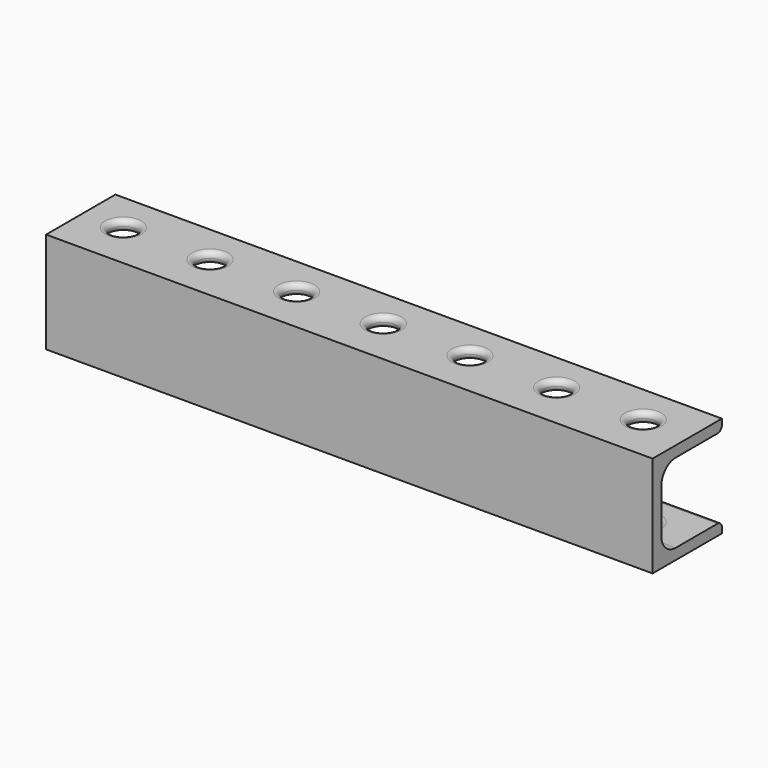
from build123d import *

# Parameters (mm, degrees)
F1_DEPTH = 168
F2_R     = 3.5
F3_DEPTH = 33
F4_R     = 5
F5_R     = 1.5
F6_R     = 1.49999
F7_R     = 1.49999
F8_R     = 1.49999


# Not quite as in the source:
# - a fillet or chamfer is up to 0.001 mm smaller than in the source, because OpenCascade refuses the exact size


with BuildPart() as f1:
    # F0 (on Right) → F1 (new body)
    with BuildSketch(Plane.YZ):
        Polygon((24, 27.9123237882), (0, 27.9123237882), (0, 0), (0, -0.0876762118), (24, -0.0876762118), (24, 2.9123237882), (3, 2.9123237882), (3, 24.9123237882), (24, 24.9123237882), align=None)
    extrude(amount=F1_DEPTH)

    # F2 (on face) → F3 (cut)
    with BuildSketch(Plane.XY.offset(27.9123237882)):
        with Locations((11, 13)):
            Circle(F2_R)
        with Locations((35, 13)):
            Circle(F2_R)
        with Locations((59, 13)):
            Circle(F2_R)
        with Locations((83, 13)):
            Circle(F2_R)
        with Locations((107, 13)):
            Circle(F2_R)
        with Locations((131, 13)):
            Circle(F2_R)
        with Locations((155, 13)):
            Circle(F2_R)
    extrude(amount=-F3_DEPTH, mode=Mode.SUBTRACT)

    # F4
    f4_edges = [f1.edges().sort_by_distance(p)[0] for p in [
        (84, 3, 24.912324),
        (84, 3, 2.912324),
    ]]
    fillet(f4_edges, radius=F4_R)

    # F5
    f5_edges = [f1.edges().sort_by_distance(p)[0] for p in [
        (84, 24, 24.912324),
        (84, 24, 2.912324),
    ]]
    fillet(f5_edges, radius=F5_R)

    # F6 (radius 1.5 in the source; OpenCascade refuses exactly that, so slightly less here)
    f6_edges = [f1.edges().sort_by_distance(p)[0] for p in [
        (7.5, 13, 27.912324),
        (7.5, 13, 24.912324),
    ]]
    fillet(f6_edges, radius=F6_R)

    # F7 (radius 1.5 in the source; OpenCascade refuses exactly that, so slightly less here)
    f7_edges = [f1.edges().sort_by_distance(p)[0] for p in [
        (31.5, 13, 24.912324),
        (31.5, 13, 27.912324),
        (55.5, 13, 24.912324),
        (55.5, 13, 27.912324),
        (79.5, 13, 24.912324),
        (79.5, 13, 27.912324),
        (103.5, 13, 24.912324),
        (103.5, 13, 27.912324),
        (127.5, 13, 24.912324),
        (127.5, 13, 27.912324),
        (151.5, 13, 24.912324),
        (151.5, 13, 27.912324),
    ]]
    fillet(f7_edges, radius=F7_R)

    # F8 (radius 1.5 in the source; OpenCascade refuses exactly that, so slightly less here)
    f8_edges = [f1.edges().sort_by_distance(p)[0] for p in [
        (7.5, 13, -0.087676),
        (7.5, 13, 2.912324),
        (31.5, 13, -0.087676),
        (31.5, 13, 2.912324),
        (55.5, 13, -0.087676),
        (55.5, 13, 2.912324),
        (79.5, 13, -0.087676),
        (79.5, 13, 2.912324),
        (103.5, 13, -0.087676),
        (103.5, 13, 2.912324),
        (127.5, 13, -0.087676),
        (127.5, 13, 2.912324),
        (151.5, 13, -0.087676),
        (151.5, 13, 2.912324),
    ]]
    fillet(f8_edges, radius=F8_R)


solid = f1.part
